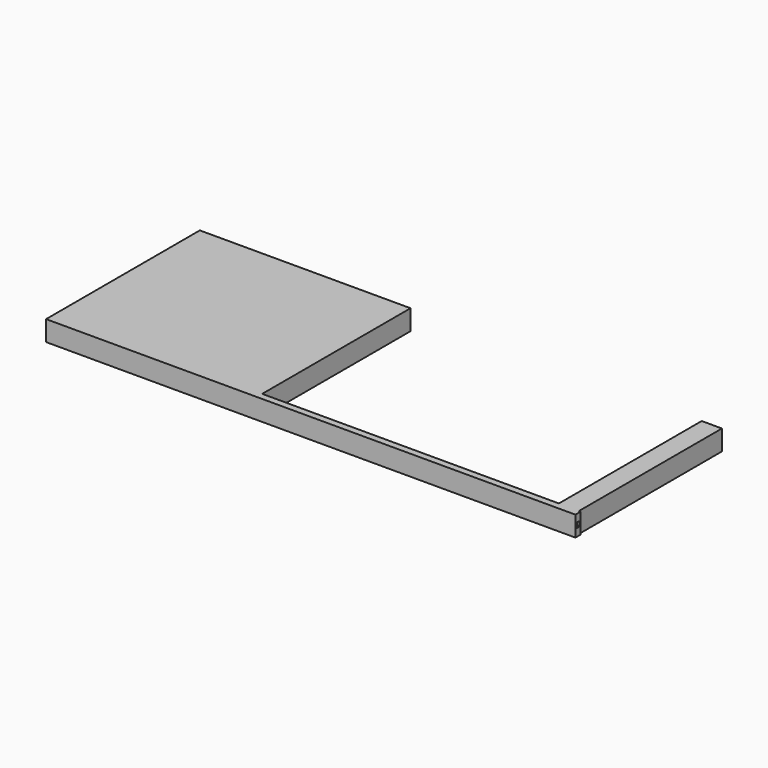
from build123d import *

# Parameters (mm, degrees)
F1_W      = 4000
F1_H      = 12000
F1_W_2    = 3400
F1_H_2    = 11400
F2_DEPTH  = 200000
F3_R      = 5475
F4_DEPTH  = 600
F5_DEPTH  = 105500
F6_DEPTH  = 12000
F8_DEPTH  = 1000
F12_W     = 12000
F12_H     = 12000
F12_R     = 5475
F13_DEPTH = 1000
F15_DEPTH = 100000
F16_W     = 3400
F16_H     = 11400
F17_DEPTH = 1000
F18_DEPTH = 300
F19_W     = 125000
F19_H     = 12000
F19_W_2   = 100000
F19_H_2   = 11400
F20_DEPTH = 110000


# Not quite as in the source:
# - the program builds the solid bodies; features that only make, move or delete a surface that nothing else refers to are left out


with BuildPart() as f2:
    # F1 (on face) → F2 (new body)
    with BuildSketch(Plane.YZ):
        Rectangle(F1_W, F1_H)
        Rectangle(F1_W_2, F1_H_2, mode=Mode.SUBTRACT)
    extrude(amount=-F2_DEPTH)

    # F3 (on face) → F4 (join)
    with BuildSketch(Plane(origin=(0, 2000, 0), x_dir=(-1, 0, 0), z_dir=(0, 1, 0))):
        with BuildLine():
            ThreePointArc((-6000, 6000), (-1757.3593128807, 4242.6406871193), (0, 0))
            Line((0, 0), (0, 6000))
            Line((0, 6000), (-6000, 6000))
        make_face()
        with BuildLine():
            ThreePointArc((-12000, 0), (-10242.6406871193, 4242.6406871193), (-6000, 6000))
            Line((-6000, 6000), (-12000, 6000))
            Line((-12000, 6000), (-12000, 0))
        make_face()
        with BuildLine():
            Line((-12000, -6000), (-6000, -6000))
            ThreePointArc((-6000, -6000), (-10242.6406871193, -4242.6406871193), (-12000, 0))
            Line((-12000, 0), (-12000, -6000))
        make_face()
        with BuildLine():
            Line((0, -6000), (0, 0))
            ThreePointArc((0, 0), (-1757.3593128807, -4242.6406871193), (-6000, -6000))
            Line((-6000, -6000), (0, -6000))
        make_face()
        with BuildLine():
            ThreePointArc((-6000, -6000), (-1757.3593128807, -4242.6406871193), (0, 0))
            ThreePointArc((0, 0), (-1757.3593128807, 4242.6406871193), (-6000, 6000))
            ThreePointArc((-6000, 6000), (-10242.6406871193, 4242.6406871193), (-12000, 0))
            ThreePointArc((-12000, 0), (-10242.6406871193, -4242.6406871193), (-6000, -6000))
        make_face()
        with Locations((-6000, 0)):
            Circle(F3_R, mode=Mode.SUBTRACT)
    extrude(amount=-F4_DEPTH)

    # F5 (add): a face of the model
    f5_faces = [f2.faces().sort_by_distance(p)[0] for p in [
        (6000, 1400, 5830.2943725152),
    ]]
    extrude(f5_faces, amount=-F5_DEPTH)

    # F6 (add): a face of the model
    f6_faces = [f2.faces().sort_by_distance(p)[0] for p in [
        (0, -300, -5875.2763053786),
    ]]
    extrude(f6_faces, amount=F6_DEPTH)

    # F7 (on face) → F8 (join)
    with BuildSketch(Plane.YZ.offset(12000)):
        with BuildLine():
            ThreePointArc((1400, 1009.9504938361), (1623.4147850968, 526.7826876426), (1700, 0))
            Line((1700, 0), (1700, 6000))
            Line((1700, 6000), (-2000, 6000))
            Line((-2000, 6000), (-2000, 0))
            ThreePointArc((-2000, 0), (-1923.4147850968, 526.7826876426), (-1700, 1009.9504938361))
            Line((-1700, 1009.9504938361), (-1700, 5700))
            Line((-1700, 5700), (1400, 5700))
            Line((1400, 5700), (1400, 1009.9504938361))
        make_face()
        with BuildLine():
            ThreePointArc((-1700, 1009.9504938361), (-150, 1850), (1400, 1009.9504938361))
            Line((1400, 1009.9504938361), (1400, 5700))
            Line((1400, 5700), (-1700, 5700))
            Line((-1700, 5700), (-1700, 1009.9504938361))
        make_face()
        with BuildLine():
            Line((1400, -5700), (1400, -1009.9504938361))
            ThreePointArc((1400, -1009.9504938361), (-150, -1850), (-1700, -1009.9504938361))
            Line((-1700, -1009.9504938361), (-1700, -5700))
            Line((-1700, -5700), (1400, -5700))
        make_face()
        with BuildLine():
            Line((1700, -6000), (1700, 0))
            ThreePointArc((1700, 0), (1623.4147850968, -526.7826876426), (1400, -1009.9504938361))
            Line((1400, -1009.9504938361), (1400, -5700))
            Line((1400, -5700), (-1700, -5700))
            Line((-1700, -5700), (-1700, -1009.9504938361))
            ThreePointArc((-1700, -1009.9504938361), (-1923.4147850968, -526.7826876426), (-2000, 0))
            Line((-2000, 0), (-2000, -6000))
            Line((-2000, -6000), (1700, -6000))
        make_face()
        with BuildLine():
            ThreePointArc((1400, -1009.9504938361), (1623.4147850968, -526.7826876426), (1700, 0))
            ThreePointArc((1700, 0), (1623.4147850968, 526.7826876426), (1400, 1009.9504938361))
            Line((1400, 1009.9504938361), (1400, 0))
            Line((1400, 0), (1400, -1009.9504938361))
        make_face()
        with BuildLine():
            Line((-1700, -3.9425e-06), (-1700, 1009.9504938361))
            ThreePointArc((-1700, 1009.9504938361), (-1923.4147850968, 526.7826876426), (-2000, 0))
            ThreePointArc((-2000, 0), (-1923.4147850968, -526.7826876426), (-1700, -1009.9504938361))
            Line((-1700, -1009.9504938361), (-1700, -3.9425e-06))
        make_face()
        with BuildLine():
            Line((1400, 0), (1400, 1009.9504938361))
            ThreePointArc((1400, 1009.9504938361), (-150, 1850), (-1700, 1009.9504938361))
            Line((-1700, 1009.9504938361), (-1700, -3.9425e-06))
            ThreePointArc((-1700, -3.9425e-06), (-150.0000019713, 1550), (1400, 0))
        make_face()
        with BuildLine():
            ThreePointArc((-1700, -1009.9504938361), (-150, -1850), (1400, -1009.9504938361))
            Line((1400, -1009.9504938361), (1400, 0))
            ThreePointArc((1400, 0), (-149.9999980287, -1550), (-1700, -3.9425e-06))
            Line((-1700, -3.9425e-06), (-1700, -1009.9504938361))
        make_face()
    extrude(amount=F8_DEPTH)

    # F12 (on face) → F13 (join)
    with BuildSketch(Plane(origin=(0, 106900, 0), x_dir=(-1, 0, 0), z_dir=(0, 1, 0))):
        with Locations((-6000, 0)):
            Rectangle(F12_W, F12_H)
        with Locations((-6000, 0)):
            Circle(F12_R, mode=Mode.SUBTRACT)
        with Locations((-6000, 0)):
            Circle(F12_R)
    extrude(amount=F13_DEPTH)

    # F14 (on face) → F15 (join)
    with BuildSketch(Plane(origin=(-200000, 0, 0), x_dir=(0, -1, 0), z_dir=(-1, 0, 0))):
        Polygon((-1700, 6000), (-1700, 5700), (1700, 5700), (1700, -5700), (-1700, -5700), (-1700, -6000), (2000, -6000), (2000, 6000), align=None)
    extrude(amount=F15_DEPTH)

    # F16 (on face) → F17 (join)
    with BuildSketch(Plane(origin=(-300000, 0, 0), x_dir=(0, -1, 0), z_dir=(-1, 0, 0))):
        Polygon((-1700, -5700), (-1700, -6000), (2000, -6000), (2000, 6000), (-1700, 6000), (-1700, 5700), (1700, 5700), (1700, -5700), align=None)
        Rectangle(F16_W, F16_H)
    extrude(amount=F17_DEPTH)

    # F18 (add): a face of the model
    f18_faces = [f2.faces().sort_by_distance(p)[0] for p in [
        (-250000, 1700, -5801.710373119),
    ]]
    extrude(f18_faces, amount=F18_DEPTH)

    # F19 (on face) → F20 (join)
    with BuildSketch(Plane(origin=(0, 2000, 0), x_dir=(-1, 0, 0), z_dir=(0, 1, 0))):
        with Locations((238500, 0)):
            Rectangle(F19_W, F19_H)
        with Locations((250000, 0)):
            Rectangle(F19_W_2, F19_H_2, mode=Mode.SUBTRACT)
    extrude(amount=F20_DEPTH)


solid = f2.part
